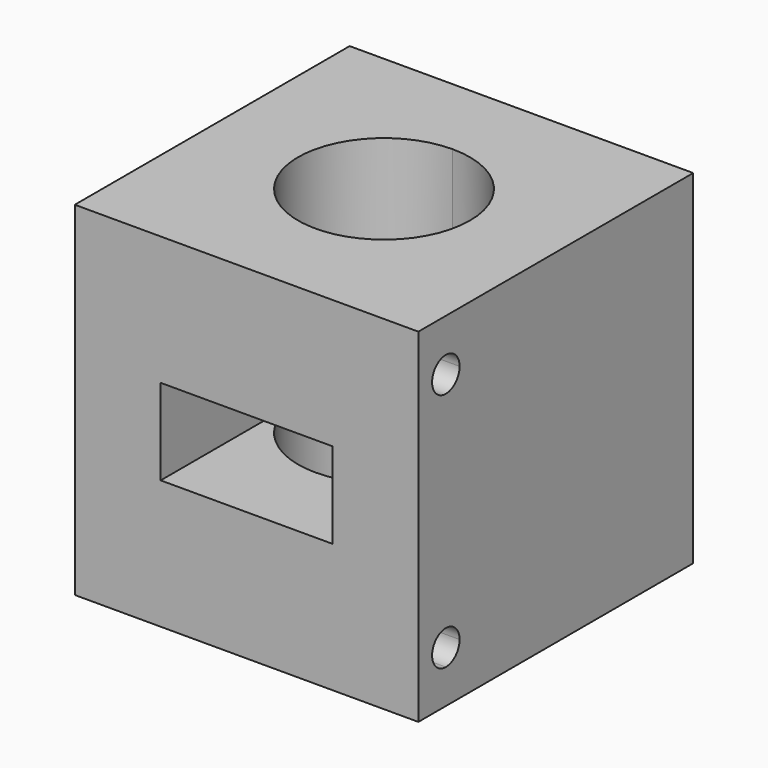
from build123d import *

# Parameters (mm, degrees)
F1_DEPTH = 25.4
F2_W     = 12.7
F2_H     = 6.35
F3_DEPTH = 25.4
F5_DEPTH = 25.4


# Not quite as in the source:
# - a feature names something its author has since deleted; it is built from what else it names


with BuildPart() as f1:
    # F0 (on Top) → F1 (new body)
    with BuildSketch(Plane.XY):
        Polygon((-3.81, 0), (0, 0), (0, 2.54), (0, 25.4), (-12.7, 25.4), (-25.4, 25.4), (-25.4, 2.54), (-25.4, 0), (-21.59, 0), align=None)
        with BuildLine():
            ThreePointArc((-6.35, 12.7), (-17.1901280605, 8.2098719395), (-12.7, 19.05))
            ThreePointArc((-12.7, 19.05), (-8.2098719395, 17.1901280605), (-6.35, 12.7))
        make_face(mode=Mode.SUBTRACT)
    extrude(amount=F1_DEPTH)

    # F2 (on face) → F3 (cut)
    with BuildSketch(Plane.XZ):
        with Locations((-12.7, 12.7)):
            Rectangle(F2_W, F2_H)
    extrude(amount=-F3_DEPTH, mode=Mode.SUBTRACT)

    # F4 (on face) → F5 (cut)
    with BuildSketch(Plane.YZ):
        with BuildLine():
            ThreePointArc((3.81, 21.59), (3.4380256121, 22.4880256121), (2.54, 22.86))
            Line((2.54, 22.86), (2.54, 21.59))
            Line((2.54, 21.59), (1.27, 21.59))
            ThreePointArc((1.27, 21.59), (2.54, 20.32), (3.81, 21.59))
        make_face()
        with BuildLine():
            Line((2.54, 21.59), (2.54, 22.86))
            ThreePointArc((2.54, 22.86), (1.6419743879, 22.4880256121), (1.27, 21.59))
            Line((1.27, 21.59), (2.54, 21.59))
        make_face()
        with BuildLine():
            ThreePointArc((3.81, 3.81), (2.54, 5.08), (1.27, 3.81))
            Line((1.27, 3.81), (2.54, 3.81))
            Line((2.54, 3.81), (2.54, 2.54))
            ThreePointArc((2.54, 2.54), (3.4380256121, 2.9119743879), (3.81, 3.81))
        make_face()
        with BuildLine():
            Line((2.54, 3.81), (1.27, 3.81))
            ThreePointArc((1.27, 3.81), (1.6419743879, 2.9119743879), (2.54, 2.54))
            Line((2.54, 2.54), (2.54, 3.81))
        make_face()
    extrude(amount=-F5_DEPTH, mode=Mode.SUBTRACT)


solid = f1.part
